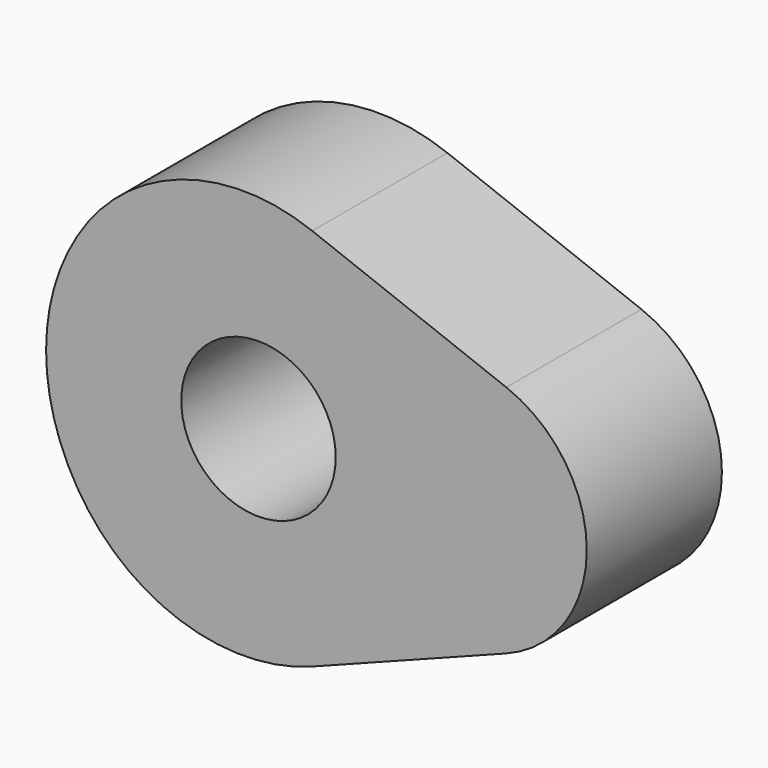
from build123d import *

# Parameters (mm, degrees)
F0_R     = 1.016
F1_DEPTH = 2.2225
F2_R     = 2.54
F3_R     = 2.54


# Not quite as in the source:
# - a length typed as a fraction of an inch, garbled in the dataset ("3 / 203.2 mm" for 3/8 in), is restored


with BuildPart() as f1:
    # F0 (on Front) → F1 (new body)
    with BuildSketch(Plane.XZ):
        with BuildLine():
            Line((3.2593966339, 1.5410604233), (0, 2.794))
            ThreePointArc((0, 2.794), (-2.794, 0), (0, -2.794))
            Line((0, -2.794), (3.2593966339, -1.5410604233))
            ThreePointArc((3.2593966339, -1.5410604233), (4.318, 0), (3.2593966339, 1.5410604233))
        make_face()
        Circle(F0_R, mode=Mode.SUBTRACT)
    extrude(amount=F1_DEPTH)

    # F2
    f2_edges = [f1.edges().sort_by_distance(p)[0] for p in [
        (0, -1.11125, 2.794),
    ]]
    fillet(f2_edges, radius=F2_R)

    # F3
    f3_edges = [f1.edges().sort_by_distance(p)[0] for p in [
        (0, -1.11125, -2.794),
    ]]
    fillet(f3_edges, radius=F3_R)


solid = f1.part
